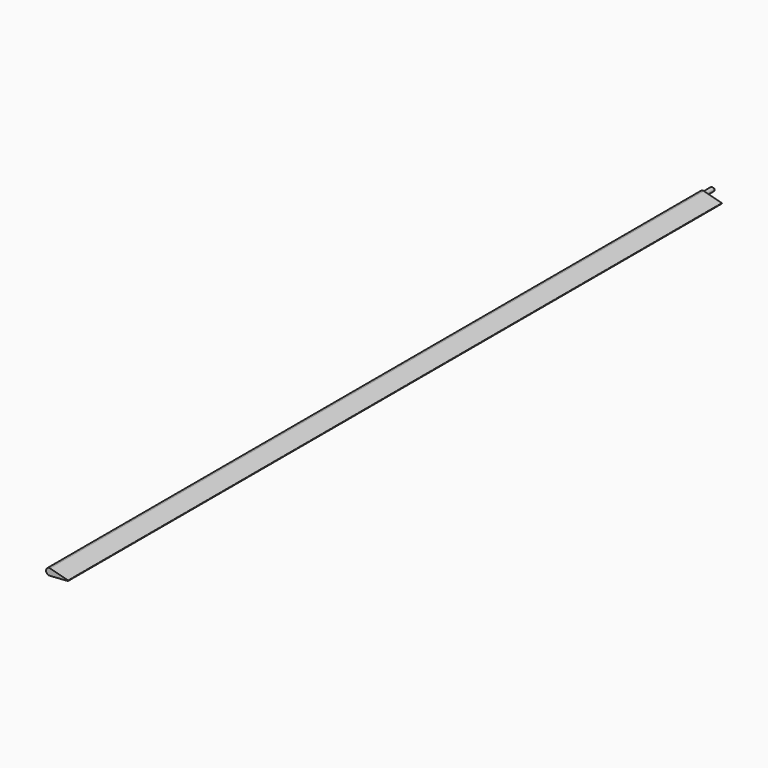
from build123d import *

# Parameters (mm, degrees)
F1_DEPTH    = 12000
F2_T1_DEPTH = 12081.8738417293
F2_T3_DEPTH = 12020.5924187821
F3_T1_DEPTH = 12151.4598397462
F4_R        = 30
F5_DEPTH    = 200
F7_DEPTH    = 50


# Not quite as in the source:
# - a fillet or chamfer that OpenCascade refuses, or shapes differently, is made with other operations: its cross-section is extruded or revolved along the edge and cut away or added


with BuildPart() as f1:
    # F0 (on Front) → F1 (new body)
    with BuildSketch(Plane.XZ):
        with BuildLine():
            Line((0, -30), (0, 50))
            ThreePointArc((0, 50), (-50, 0), (0, -50))
            Line((0, -50), (0, -30))
        make_face()
        Polygon((300, -30), (0, 50), (0, -30), align=None)
        Polygon((300, -30), (0, -30), (0, -50), align=None)
    extrude(amount=F1_DEPTH)

    # F2: fillet of radius 40 on 2 edges, made by hand

    # F2_s2 → F2_t1 (cut)
    with BuildSketch(Plane.XZ.offset(-40.9369208646)):
        with BuildLine():
            ThreePointArc((7.0757568477, 48.1131315073), (-4.5979720129, 49.4403608659), (-16.1537458737, 47.3186696162))
            ThreePointArc((-16.1537458737, 47.3186696162), (-8.1873841729, 49.325112675), (0, 50))
            Line((0, 50), (7.0757568477, 48.1131315073))
        make_face()
    extrude(amount=F2_T1_DEPTH, mode=Mode.SUBTRACT)

    # F2_s4 → F2_t3 (cut)
    with BuildSketch(Plane.XZ.offset(-10.296209391)):
        with BuildLine():
            ThreePointArc((-4.1149894068, -49.8303809155), (-1.1394908774, -49.9648240658), (1.8377625396, -49.8774824974))
            Line((1.8377625396, -49.8774824974), (0, -50))
            ThreePointArc((0, -50), (-2.0592418782, -49.957577232), (-4.1149894068, -49.8303809155))
        make_face()
    extrude(amount=F2_T3_DEPTH, mode=Mode.SUBTRACT)

    # F3: fillet of radius 5 on 1 edges, made by hand

    # F3_s2 → F3_t1 (cut)
    with BuildSketch(Plane.XZ.offset(-75.7299198731)):
        with BuildLine():
            ThreePointArc((270.7308421782, -22.1948912475), (274.4190165752, -27.51039091), (269.775123978, -32.0149917348))
            Line((269.775123978, -32.0149917348), (300, -30))
            Line((300, -30), (270.7308421782, -22.1948912475))
        make_face()
    extrude(amount=F3_T1_DEPTH, mode=Mode.SUBTRACT)

    # F4 (on Front) → F5 (join)
    with BuildSketch(Plane.XZ):
        Circle(F4_R)
    extrude(amount=-F5_DEPTH)

    # F6 (on Top) → F7 (cut, symmetric)
    with BuildSketch(Plane.XY):
        with BuildLine():
            ThreePointArc((0, 160), (28.2842712475, 171.7157287525), (40, 200))
            ThreePointArc((40, 200), (-28.2842712475, 228.2842712475), (0, 160))
        make_face()
    extrude(amount=F7_DEPTH, both=True, mode=Mode.SUBTRACT)


solid = f1.part
